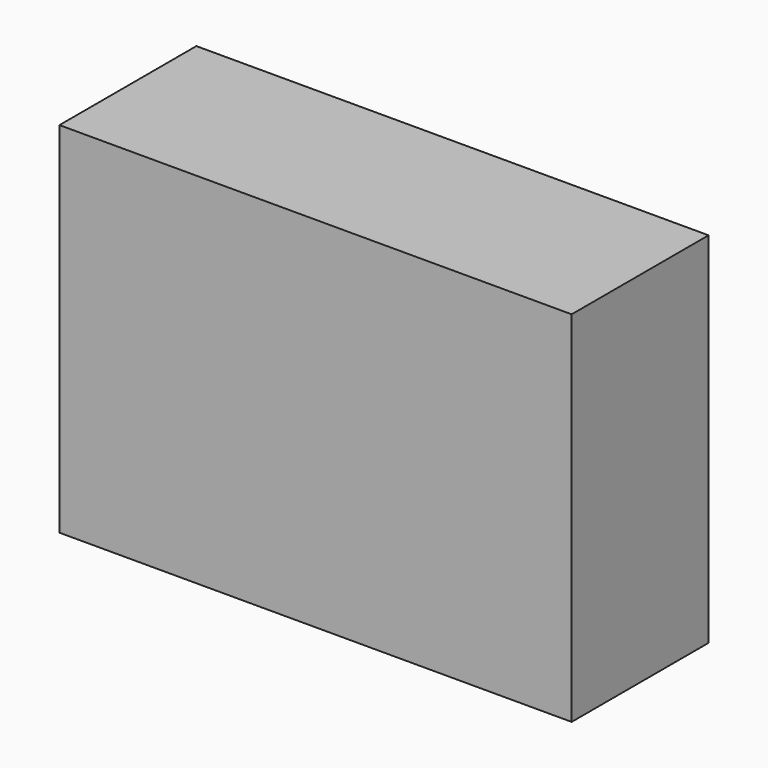
from build123d import *

# Parameters (mm, degrees)
F0_W         = 76.0295242071
F0_H         = 53.2652959228
F1_DEPTH     = 25.4
F2_TEXT_SIZE = 16.54202222
F3_DEPTH     = 25.4


# Not quite as in the source:
# - Text() gives the source's letters only with a copy of the font that has no kerning and outlines rounded to 1/6400 em; it was checked with that copy


with BuildPart() as f1:
    # F0 (on Front) → F1 (new body)
    with BuildSketch(Plane.XZ):
        with Locations((38.0147621036, 26.6326479614)):
            Rectangle(F0_W, F0_H)
    extrude(amount=F1_DEPTH)

    # F2 (on Front) → F3 (join)
    with BuildSketch(Plane.XZ):
        with Locations((2.8441837057, 36.1149571836)):
            Text('Declan', F2_TEXT_SIZE, font='Open Sans', text_align=(TextAlign.LEFT, TextAlign.BOTTOM))
    extrude(amount=F3_DEPTH)


solid = f1.part
